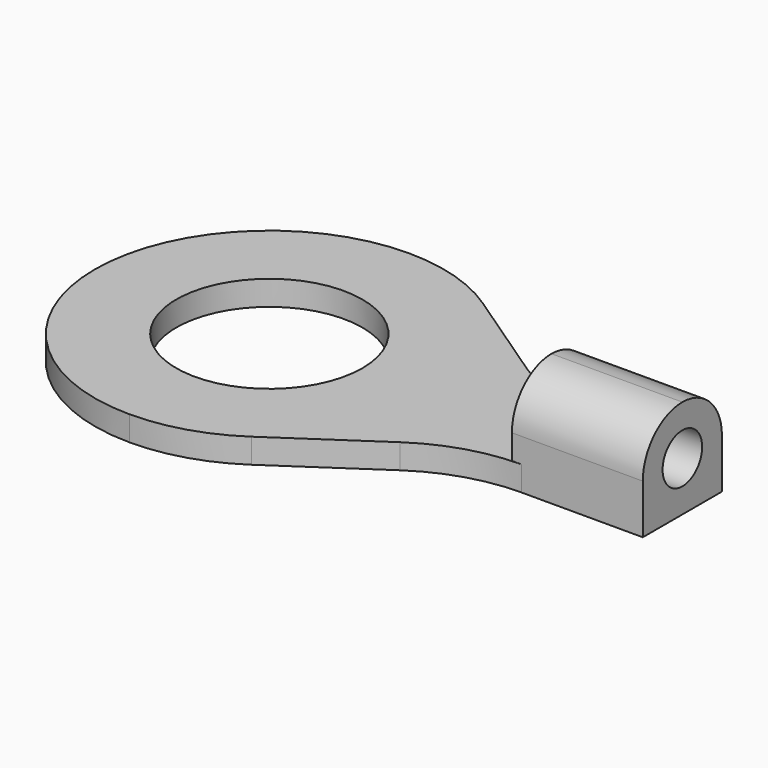
from build123d import *

# Parameters (mm, degrees)
F0_R     = 3.2
F1_DEPTH = 0.85
F3_DEPTH = 2.55
F4_R     = 1.69999
F5_R     = 0.85
F6_DEPTH = 25


# Not quite as in the source:
# - a fillet or chamfer is up to 0.001 mm smaller than in the source, because OpenCascade refuses the exact size


with BuildPart() as f1:
    # F0 (on Top) → F1 (new body)
    with BuildSketch(Plane.XY):
        with BuildLine():
            Line((16.0373335058, 4.3), (20.2, 4.3))
            Line((20.2, 4.3), (20.2, 7.7))
            Line((20.2, 7.7), (16.0373335058, 7.7))
            ThreePointArc((16.0373335058, 7.7), (14.2805243712, 7.9629605488), (12.6777057346, 8.7287927785))
            Line((12.6777057346, 8.7287927785), (9.3596277711, 10.9712072215))
            ThreePointArc((9.3596277711, 10.9712072215), (7.7568091346, 11.7370394512), (6, 12))
            ThreePointArc((6, 12), (1.7573593129, 10.2426406871), (0, 6))
            ThreePointArc((0, 6), (1.7573593129, 1.7573593129), (6, 0))
            ThreePointArc((6, 0), (7.7568091346, 0.2629605488), (9.3596277711, 1.0287927785))
            Line((9.3596277711, 1.0287927785), (12.6777057346, 3.2712072215))
            ThreePointArc((12.6777057346, 3.2712072215), (14.2805243712, 4.0370394512), (16.0373335058, 4.3))
        make_face()
        with Locations((6, 6)):
            Circle(F0_R, mode=Mode.SUBTRACT)
    extrude(amount=F1_DEPTH)

    # F2 (on face) → F3 (join)
    with BuildSketch(Plane.XY.offset(0.85)):
        Polygon((20.2, 4.3), (20.2, 7.7), (16.0373335058, 7.7), (15.7, 7.7), (15.7, 4.3), (16.0373335058, 4.3), align=None)
    extrude(amount=F3_DEPTH)

    # F4 (radius 1.7 in the source; OpenCascade refuses exactly that, so slightly less here)
    f4_edges = [f1.edges().sort_by_distance(p)[0] for p in [
        (17.95, 7.7, 3.4),
        (17.95, 4.3, 3.4),
    ]]
    fillet(f4_edges, radius=F4_R)

    # F5 (on face) → F6 (cut)
    with BuildSketch(Plane.YZ.offset(20.2)):
        with Locations((6, 1.7)):
            Circle(F5_R)
    extrude(amount=-F6_DEPTH, mode=Mode.SUBTRACT)


solid = f1.part
